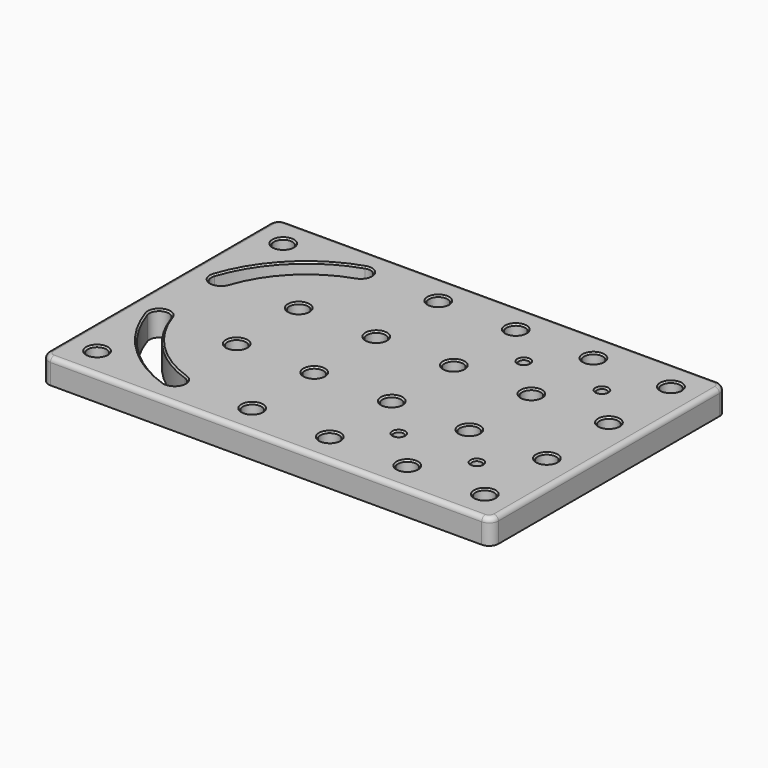
from build123d import *

# Parameters (mm, degrees)
F0_W         = 145
F0_H         = 95
F0_R         = 3
F0_R_2       = 1.6
F1_DEPTH     = 8
F2_R         = 1.5
F3_SIZE      = 0.5
F4_T1_DEPTH  = 15.5
F4_T4_ANGLE  = 90
F4_T6_ANGLE  = 90
F4_T8_ANGLE  = 90
F4_T10_ANGLE = 90


# Not quite as in the source:
# - a fillet or chamfer that OpenCascade refuses, or shapes differently, is made with other operations: its cross-section is extruded or revolved along the edge and cut away or added
# - a feature names something its author has since deleted; it is built from what else it names


with BuildPart() as f1:
    # F0 (on Top) → F1 (new body)
    with BuildSketch(Plane.XY):
        with Locations((-44.7653323412, -10.0623860955)):
            Rectangle(F0_W, F0_H)
        with Locations((-107.2653323412, -47.5623860955)):
            Circle(F0_R, mode=Mode.SUBTRACT)
        with BuildLine():
            ThreePointArc((-83.2614498041, -50.5507384844), (-99.9435684207, -40.240622175), (-110.2536847301, -23.5585035585))
            ThreePointArc((-110.2536847301, -23.5585035585), (-108.2614498041, -19.5740337067), (-104.2769799523, -21.5662686326))
            ThreePointArc((-104.2769799523, -21.5662686326), (-95.4887956992, -35.7858494535), (-81.2692148782, -44.5740337067))
            ThreePointArc((-81.2692148782, -44.5740337067), (-79.2769799523, -48.5585035585), (-83.2614498041, -50.5507384844))
        make_face(mode=Mode.SUBTRACT)
        with Locations((-57.2653323412, -47.5623860955)):
            Circle(F0_R, mode=Mode.SUBTRACT)
        with Locations((-82.2653323412, -22.5623860955)):
            Circle(F0_R, mode=Mode.SUBTRACT)
        with Locations((-57.2653323412, -22.5623860955)):
            Circle(F0_R, mode=Mode.SUBTRACT)
        with Locations((-32.2653323412, -47.5623860955)):
            Circle(F0_R, mode=Mode.SUBTRACT)
        with Locations((-19.8653323412, -35.2623860955)):
            Circle(F0_R_2, mode=Mode.SUBTRACT)
        with Locations((-7.2653323412, -47.5623860955)):
            Circle(F0_R, mode=Mode.SUBTRACT)
        with Locations((17.7346676588, -47.5623860955)):
            Circle(F0_R, mode=Mode.SUBTRACT)
        with Locations((5.3346676588, -35.2623860955)):
            Circle(F0_R_2, mode=Mode.SUBTRACT)
        with Locations((-32.2653323412, -22.5623860955)):
            Circle(F0_R, mode=Mode.SUBTRACT)
        with Locations((-7.2653323412, -22.5623860955)):
            Circle(F0_R, mode=Mode.SUBTRACT)
        with Locations((17.7346676588, -22.5623860955)):
            Circle(F0_R, mode=Mode.SUBTRACT)
        with Locations((-82.2653323412, 2.4376139045)):
            Circle(F0_R, mode=Mode.SUBTRACT)
        with Locations((-57.2653323412, 2.4376139045)):
            Circle(F0_R, mode=Mode.SUBTRACT)
        with BuildLine():
            ThreePointArc((-110.2536847301, 3.4337313674), (-99.9435684207, 20.115849984), (-83.2614498041, 30.4259662933))
            ThreePointArc((-83.2614498041, 30.4259662933), (-79.2769799523, 28.4337313674), (-81.2692148782, 24.4492615156))
            ThreePointArc((-81.2692148782, 24.4492615156), (-95.4887956992, 15.6610772625), (-104.2769799523, 1.4414964415))
            ThreePointArc((-104.2769799523, 1.4414964415), (-108.2614498041, -0.5507384844), (-110.2536847301, 3.4337313674))
        make_face(mode=Mode.SUBTRACT)
        with Locations((-107.2653323412, 27.4376139045)):
            Circle(F0_R, mode=Mode.SUBTRACT)
        with Locations((-57.2653323412, 27.4376139045)):
            Circle(F0_R, mode=Mode.SUBTRACT)
        with Locations((-32.2653323412, 2.4376139045)):
            Circle(F0_R, mode=Mode.SUBTRACT)
        with Locations((-7.2653323412, 2.4376139045)):
            Circle(F0_R, mode=Mode.SUBTRACT)
        with Locations((17.7346676588, 2.4376139045)):
            Circle(F0_R, mode=Mode.SUBTRACT)
        with Locations((-19.8653323412, 15.1376139045)):
            Circle(F0_R_2, mode=Mode.SUBTRACT)
        with Locations((-32.2653323412, 27.4376139045)):
            Circle(F0_R, mode=Mode.SUBTRACT)
        with Locations((5.3346676588, 15.1376139045)):
            Circle(F0_R_2, mode=Mode.SUBTRACT)
        with Locations((-7.2653323412, 27.4376139045)):
            Circle(F0_R, mode=Mode.SUBTRACT)
        with Locations((17.7346676588, 27.4376139045)):
            Circle(F0_R, mode=Mode.SUBTRACT)
    extrude(amount=-F1_DEPTH)

    # F2
    f2_edges = [f1.edges().sort_by_distance(p)[0] for p in [
        (-117.265332, -10.062386, 0),
        (-44.765332, 37.437614, 0),
        (-44.765332, -57.562386, 0),
        (27.734668, -10.062386, 0),
    ]]
    fillet(f2_edges, radius=F2_R)

    # F3
    f3_edges = [f1.edges().sort_by_distance(p)[0] for p in [
        (-115.765332, -10.062386, 0),
        (-44.765332, 35.937614, 0),
        (-44.765332, -56.062386, 0),
        (26.234668, -10.062386, 0),
        (-110.265332, -47.562386, 0),
        (-95.488796, -35.785849, 0),
        (-79.27698, -48.558504, 0),
        (-99.943568, -40.240622, 0),
        (-108.26145, -19.574034, 0),
        (-60.265332, -47.562386, 0),
        (-85.265332, -22.562386, 0),
        (-60.265332, -22.562386, 0),
        (-35.265332, -47.562386, 0),
        (-21.465332, -35.262386, 0),
        (-10.265332, -47.562386, 0),
        (14.734668, -47.562386, 0),
        (3.734668, -35.262386, 0),
        (-35.265332, -22.562386, 0),
        (-10.265332, -22.562386, 0),
        (14.734668, -22.562386, 0),
        (-85.265332, 2.437614, 0),
        (-60.265332, 2.437614, 0),
        (-99.943568, 20.11585, 0),
        (-79.27698, 28.433731, 0),
        (-95.488796, 15.661077, 0),
        (-108.26145, -0.550738, 0),
        (-110.265332, 27.437614, 0),
        (-60.265332, 27.437614, 0),
        (-35.265332, 2.437614, 0),
        (-10.265332, 2.437614, 0),
        (14.734668, 2.437614, 0),
        (-21.465332, 15.137614, 0),
        (-35.265332, 27.437614, 0),
        (3.734668, 15.137614, 0),
        (-10.265332, 27.437614, 0),
        (14.734668, 27.437614, 0),
    ]]
    chamfer(f3_edges, length=F3_SIZE)

    # F4: fillet of radius 3 on 4 edges, made by hand

    # F4_s2 → F4_t1 (cut)
    with BuildSketch(Plane.XY.offset(-15.5)):
        with BuildLine():
            ThreePointArc((-117.2653323412, -54.5623860955), (-116.3866526848, -56.6837064391), (-114.2653323412, -57.5623860955))
            Line((-114.2653323412, -57.5623860955), (-117.2653323412, -57.5623860955))
            Line((-117.2653323412, -57.5623860955), (-117.2653323412, -54.5623860955))
        make_face()
        with BuildLine():
            ThreePointArc((24.7346676588, -57.5623860955), (26.8559880024, -56.6837064391), (27.7346676588, -54.5623860955))
            Line((27.7346676588, -54.5623860955), (27.7346676588, -57.5623860955))
            Line((27.7346676588, -57.5623860955), (24.7346676588, -57.5623860955))
        make_face()
        with BuildLine():
            ThreePointArc((24.7346676588, 37.4376139045), (26.8559880024, 36.558934248), (27.7346676588, 34.4376139045))
            Line((27.7346676588, 34.4376139045), (27.7346676588, 37.4376139045))
            Line((27.7346676588, 37.4376139045), (24.7346676588, 37.4376139045))
        make_face()
        with BuildLine():
            ThreePointArc((-117.2653323412, 34.4376139045), (-116.3866526848, 36.558934248), (-114.2653323412, 37.4376139045))
            Line((-114.2653323412, 37.4376139045), (-117.2653323412, 37.4376139045))
            Line((-117.2653323412, 37.4376139045), (-117.2653323412, 34.4376139045))
        make_face()
    extrude(amount=F4_T1_DEPTH, mode=Mode.SUBTRACT)

    # F4_s3 → F4_t4 (revolve, cut)
    with BuildSketch(Plane.YZ.offset(-114.2653323412)):
        with BuildLine():
            ThreePointArc((35.9376139045, 0), (36.9982740763, -0.4393398282), (37.4376139045, -1.5))
            Line((37.4376139045, -1.5), (37.4376139045, 0))
            Line((37.4376139045, 0), (35.9376139045, 0))
        make_face()
    revolve(axis=Axis((-114.2653323412, 34.4376139045, 0), (0, 0, 1)), revolution_arc=F4_T4_ANGLE, mode=Mode.SUBTRACT)

    # F4_s5 → F4_t6 (revolve, cut)
    with BuildSketch(Plane.XZ.offset(-34.4376139045)):
        with BuildLine():
            ThreePointArc((26.2346676588, 0), (27.2953278306, -0.4393398282), (27.7346676588, -1.5))
            Line((27.7346676588, -1.5), (27.7346676588, 0))
            Line((27.7346676588, 0), (26.2346676588, 0))
        make_face()
    revolve(axis=Axis((24.7346676588, 34.4376139045, 0), (0, 0, 1)), revolution_arc=F4_T6_ANGLE, mode=Mode.SUBTRACT)

    # F4_s7 → F4_t8 (revolve, cut)
    with BuildSketch(Plane.YZ.offset(24.7346676588)):
        with BuildLine():
            ThreePointArc((-56.0623860955, 0), (-57.1230462673, -0.4393398282), (-57.5623860955, -1.5))
            Line((-57.5623860955, -1.5), (-57.5623860955, 0))
            Line((-57.5623860955, 0), (-56.0623860955, 0))
        make_face()
    revolve(axis=Axis((24.7346676588, -54.5623860955, 0), (0, 0, 1)), revolution_arc=F4_T8_ANGLE, mode=Mode.SUBTRACT)

    # F4_s9 → F4_t10 (revolve, cut)
    with BuildSketch(Plane.XZ.offset(54.5623860955)):
        with BuildLine():
            ThreePointArc((-115.7653323412, 0), (-116.825992513, -0.4393398282), (-117.2653323412, -1.5))
            Line((-117.2653323412, -1.5), (-117.2653323412, 0))
            Line((-117.2653323412, 0), (-115.7653323412, 0))
        make_face()
    revolve(axis=Axis((-114.2653323412, -54.5623860955, 0), (0, 0, 1)), revolution_arc=F4_T10_ANGLE, mode=Mode.SUBTRACT)


solid = f1.part
